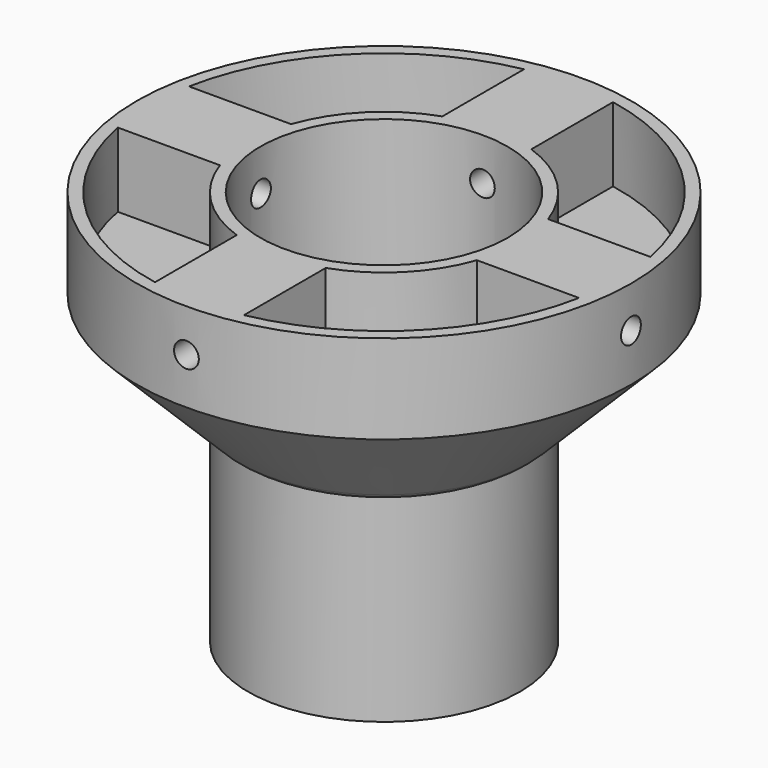
from build123d import *

# Parameters (mm, degrees)
F0_R     = 31.75
F0_R_2   = 17.4625
F1_DEPTH = 25.4
F0_R_3   = 15.875
F2_DEPTH = 50.8
F3_SIZE  = 13.97
F6_DEPTH = 9.525
F10_D    = 3.175
F13_D    = 3.175


# Not quite as in the source:
# - a fillet or chamfer that OpenCascade refuses, or shapes differently, is made with other operations: its cross-section is extruded or revolved along the edge and cut away or added


with BuildPart() as f1:
    # F0 (on Top) → F1 (new body)
    with BuildSketch(Plane.XY):
        Circle(F0_R)
        Circle(F0_R_2, mode=Mode.SUBTRACT)
    extrude(amount=-F1_DEPTH)

    # F0 (on Top) → F2 (join)
    with BuildSketch(Plane.XY):
        Circle(F0_R_2)
        Circle(F0_R_3, mode=Mode.SUBTRACT)
    extrude(amount=-F2_DEPTH)

    # F3
    f3_edges = [f1.edges().sort_by_distance(p)[0] for p in [
        (-31.75, 0, -25.4),
    ]]
    chamfer(f3_edges, length=F3_SIZE)

    # F4: fillet of radius 5.08 on 1 edges, made by hand

    # F4_s1 → F4_t2 (revolve, cut)
    with BuildSketch(Plane.XZ):
        with BuildLine():
            ThreePointArc((18.677323371, -24.502676629), (18.1034449464, -24.9967366519), (17.4625, -25.4))
            Line((17.4625, -25.4), (17.78, -25.4))
            Line((17.78, -25.4), (18.677323371, -24.502676629))
        make_face()
    revolve(axis=Axis((0, 0, -25.4), (0, 0, 1)), mode=Mode.SUBTRACT)

    # F5 (on Top) → F6 (cut)
    with BuildSketch(Plane.XY):
        with BuildLine():
            ThreePointArc((-5.715, 29.6161304233), (-21.3281082875, 21.3281082875), (-29.6161304233, 5.715))
            Line((-29.6161304233, 5.715), (-16.5008388044, 5.715))
            ThreePointArc((-16.5008388044, 5.715), (-12.3478521665, 12.3478521665), (-5.715, 16.5008388044))
            Line((-5.715, 16.5008388044), (-5.715, 29.6161304233))
        make_face()
        with BuildLine():
            ThreePointArc((-29.6161304233, -5.715), (-21.3281082875, -21.3281082875), (-5.715, -29.6161304233))
            Line((-5.715, -29.6161304233), (-5.715, -16.5008388044))
            ThreePointArc((-5.715, -16.5008388044), (-12.3478521665, -12.3478521665), (-16.5008388044, -5.715))
            Line((-16.5008388044, -5.715), (-29.6161304233, -5.715))
        make_face()
        with BuildLine():
            Line((5.715, -16.5008388044), (5.715, -29.6161304233))
            ThreePointArc((5.715, -29.6161304233), (21.3281082875, -21.3281082875), (29.6161304233, -5.715))
            Line((29.6161304233, -5.715), (16.5008388044, -5.715))
            ThreePointArc((16.5008388044, -5.715), (12.3478521665, -12.3478521665), (5.715, -16.5008388044))
        make_face()
        with BuildLine():
            Line((16.5008388044, 5.715), (29.6161304233, 5.715))
            ThreePointArc((29.6161304233, 5.715), (21.3281082875, 21.3281082875), (5.715, 29.6161304233))
            Line((5.715, 29.6161304233), (5.715, 16.5008388044))
            ThreePointArc((5.715, 16.5008388044), (12.3478521665, 12.3478521665), (16.5008388044, 5.715))
        make_face()
    extrude(amount=-F6_DEPTH, mode=Mode.SUBTRACT)

    # F10 (through all)
    with Locations(Plane.XZ.offset(50.8)):
        with Locations((0, -5.4679759778)):
            Hole(F10_D / 2)

    # F13 (through all)
    with Locations(Plane.YZ.offset(50.8)):
        with Locations((0, -5.3200940602)):
            Hole(F13_D / 2)


solid = f1.part
